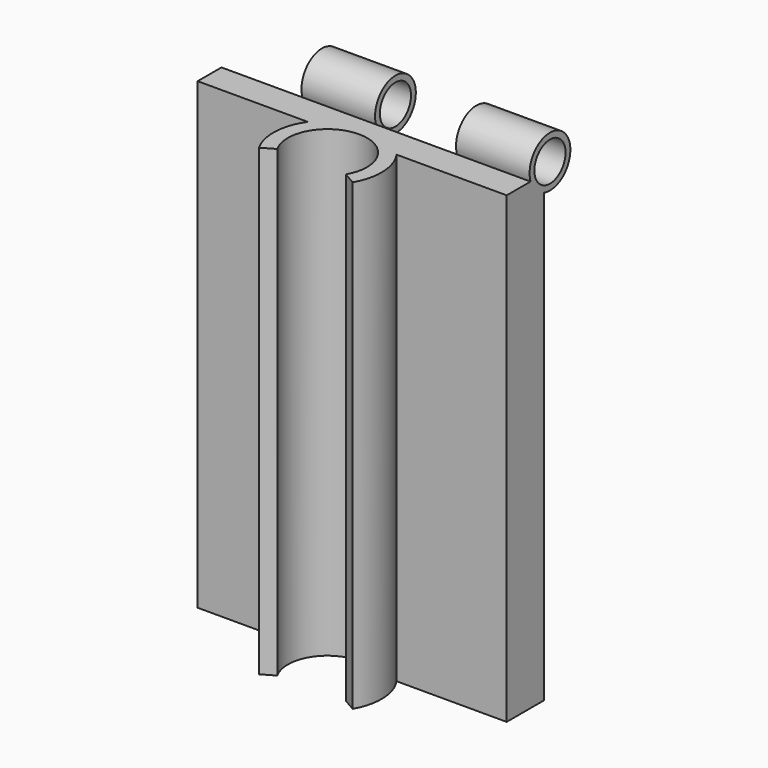
from build123d import *

# Parameters (mm, degrees)
F0_W          = 127
F0_H          = 190.5
F1_DEPTH      = 9.525
F3_DEPTH      = 95.251
F3_DEPTH_BACK = 95.251
F4_DEPTH      = 95.25
F5_R          = 10.4775
F5_R_2        = 8.001
F6_DEPTH      = 63.501
F6_DEPTH_BACK = 63.501
F7_DEPTH      = 30.226
F8_R          = 10.4775
F8_R_2        = 8.001
F9_DEPTH      = 30.226


# Not quite as in the source:
# - a pattern or mirror of a feature is missing from the dataset's text; its kind, count and spacing are read off the source's solid


with BuildPart() as f1:
    # F0 (on Front) → F1 (new body, symmetric)
    with BuildSketch(Plane.XZ):
        Rectangle(F0_W, F0_H)
    extrude(amount=F1_DEPTH, both=True)

    # F2 (on Top) → F3 (cut, two sides)
    with BuildSketch(Plane.XY) as f3_sk:
        with BuildLine():
            Line((14.0918571172, -30.3609375), (19.2474145991, -33.3375))
            ThreePointArc((19.2474145991, -33.3375), (0, 0), (-19.2474145991, -33.3375))
            Line((-19.2474145991, -33.3375), (-14.0918571172, -30.3609375))
            ThreePointArc((-14.0918571172, -30.3609375), (0, -5.953125), (14.0918571172, -30.3609375))
        make_face()
        with BuildLine():
            Line((0, -22.225), (14.0918571172, -30.3609375))
            ThreePointArc((14.0918571172, -30.3609375), (0, -5.953125), (-14.0918571172, -30.3609375))
            Line((-14.0918571172, -30.3609375), (0, -22.225))
        make_face()
    extrude(amount=F3_DEPTH, mode=Mode.SUBTRACT)
    extrude(f3_sk.sketch, amount=-F3_DEPTH_BACK, mode=Mode.SUBTRACT)

    # F2 (on Top) → F4 (join, symmetric)
    with BuildSketch(Plane.XY):
        with BuildLine():
            Line((14.0918571172, -30.3609375), (19.2474145991, -33.3375))
            ThreePointArc((19.2474145991, -33.3375), (0, 0), (-19.2474145991, -33.3375))
            Line((-19.2474145991, -33.3375), (-14.0918571172, -30.3609375))
            ThreePointArc((-14.0918571172, -30.3609375), (0, -5.953125), (14.0918571172, -30.3609375))
        make_face()
    extrude(amount=F4_DEPTH, both=True)

    # F5 (on Right) → F6 (cut, two sides)
    with BuildSketch(Plane.YZ) as f6_sk:
        with Locations((12.7, 98.425)):
            Circle(F5_R)
        with Locations((12.7, 98.425)):
            Circle(F5_R_2, mode=Mode.SUBTRACT)
        with Locations((12.7, 98.425)):
            Circle(F5_R_2)
    extrude(amount=-F6_DEPTH, mode=Mode.SUBTRACT)
    extrude(f6_sk.sketch, amount=F6_DEPTH_BACK, mode=Mode.SUBTRACT)

    # F5 (on Right) → F7 (join)
    with BuildSketch(Plane.YZ):
        with Locations((12.7, 98.425)):
            Circle(F5_R)
        with Locations((12.7, 98.425)):
            Circle(F5_R_2, mode=Mode.SUBTRACT)
    f7 = extrude(amount=-F7_DEPTH)

    # F7_copies: F7 across plane
    add(f7.mirror(Plane(origin=(16.637, 0, 0), x_dir=(0, 0, 1), z_dir=(1, 0, 0))))

    # F8 (on face) → F9 (join)
    with BuildSketch(Plane.YZ):
        with Locations((12.7, 98.425)):
            Circle(F8_R)
        with Locations((12.7, 98.425)):
            Circle(F8_R_2, mode=Mode.SUBTRACT)
    extrude(amount=-F9_DEPTH)


solid = f1.part
